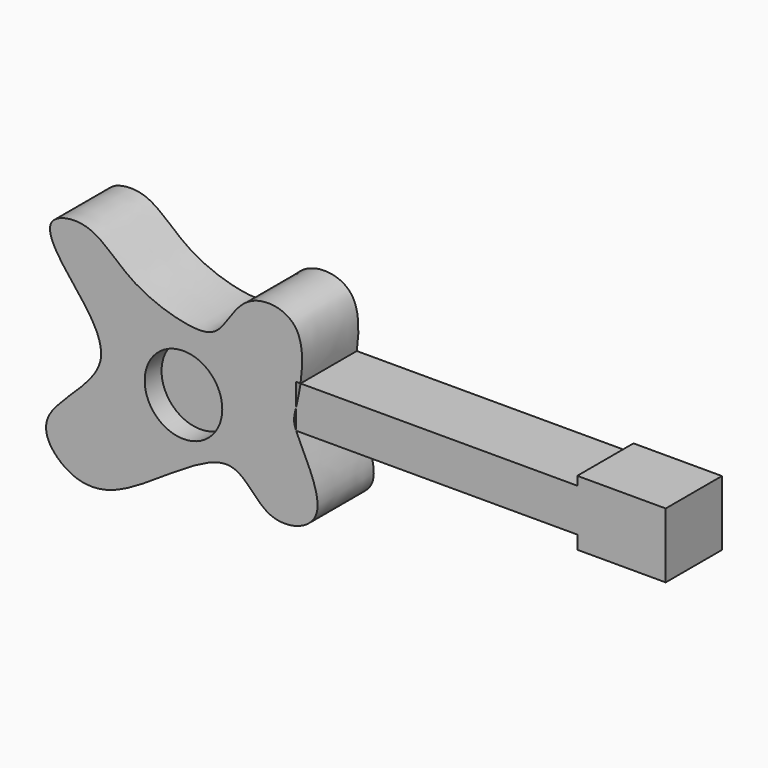
from build123d import *

# Parameters (mm, degrees)
F1_DEPTH = 12.7
F2_R     = 7.0092293816
F3_DEPTH = 3.81


with BuildPart() as f1:
    # F0 (on Front) → F1 (new body)
    with BuildSketch(Plane.XZ):
        with BuildLine():
            add(Edge.make_bspline(
                [(0.8029544839, 4.0648496944), (1.2347652941, 7.0241145987), (1.4721495297, 14.7996883678), (-9.6708628109, 15.9878996128), (-13.284612676, 7.1356193282), (-18.6542603724, 6.0613556173), (-30.3426752266, 9.6016721768), (-36.6529788005, 17.8275013443), (-46.2444318253, 15.9160192782), (-42.1270089818, 7.9260424689), (-29.7108350462, -4.5676802797), (-47.6417812778, -15.0925906587), (-43.1936717702, -23.3534478137), (-32.4283903553, -27.2234215927), (-11.4506857343, -7.1683016979), (-6.0701150443, -21.2321567841), (7.8820914243, -17.1243085579), (1.0747376663, -6.4765977067), (0, -3.7123864744)],
                knots=[0.023269045, 0.023269045, 0.023269045, 0.023269045, 0.0667571713, 0.1218537224, 0.1761755653, 0.2172246557, 0.2818209165, 0.3423178482, 0.3897205506, 0.4392457667, 0.5104721831, 0.5842367479, 0.6322613056, 0.6915883027, 0.7828764166, 0.8412193089, 0.8966720426, 0.9636486809, 0.9636486809, 0.9636486809, 0.9636486809], degree=3))
            add(Edge.make_bspline(
                [(0, -3.7123864744), (-0.5833098349, -2.2121212021), (-0.3862011269, -1.6134754239), (0, 0)],
                knots=[0.9636486809, 0.9636486809, 0.9636486809, 0.9636486809, 1, 1, 1, 1], degree=3))
            Line((0, 0), (0, 4.0648496944))
            Line((0, 4.0648496944), (0.8029544839, 4.0648496944))
        make_face()
    extrude(amount=F1_DEPTH)

    # F2 (on face) → F3 (cut)
    with BuildSketch(Plane.XZ.offset(12.7)):
        with Locations((-20.3506015241, -4.6396516263)):
            Circle(F2_R)
    extrude(amount=-F3_DEPTH, mode=Mode.SUBTRACT)


with BuildPart() as f1b:
    # F0 (on Front) → F1, piece 2 (new body)
    with BuildSketch(Plane.XZ):
        with BuildLine():
            Line((0, 0), (0, -3.7123864744))
            Line((0, -3.7123864744), (50.8, -3.7123864744))
            Line((50.8, -3.7123864744), (50.8, 4.0648496944))
            Line((50.8, 4.0648496944), (0.8029544839, 4.0648496944))
            add(Edge.make_bspline(
                [(0, 0), (0.2472133512, 1.0328107271), (0.5719069301, 2.4814458031), (0.8029544839, 4.0648496944)],
                knots=[0, 0, 0, 0, 0.023269045, 0.023269045, 0.023269045, 0.023269045], degree=3))
        make_face()
        Polygon((50.8, 4.0648496944), (50.8, -3.7123864744), (50.8, -6.126340013), (66.7771026492, -6.126340013), (66.7771026492, 5.6362333708), (50.8, 5.6362333708), align=None)
    extrude(amount=F1_DEPTH)


solid = Compound([f1.part, f1b.part])
